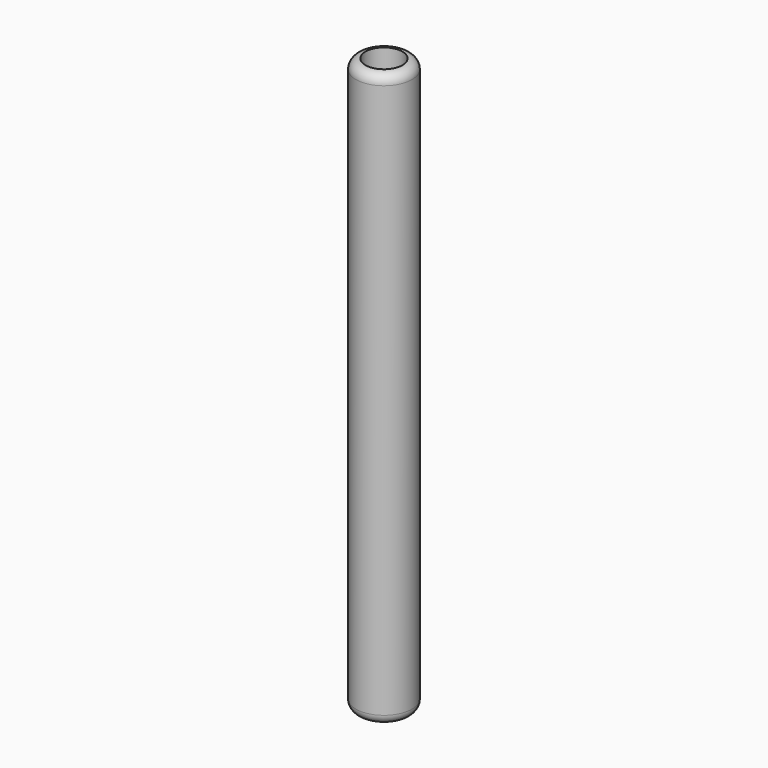
from build123d import *

# Parameters (mm, degrees)
F0_W    = 2.54
F0_H    = 152.4
F2_F1_R = 2.5399
F2_F2_R = 2.5399


# Not quite as in the source:
# - a fillet or chamfer is up to 0.001 mm smaller than in the source, because OpenCascade refuses the exact size


with BuildPart() as f1:
    # F0 (on Front) → F1 (revolve)
    with BuildSketch(Plane.XZ):
        with Locations((-6.1784988933, 0.9033400565)):
            Rectangle(F0_W, F0_H)
    revolve(axis=Axis((0, 0, -1.1060908437), (0, 0, 1)))

    # F2: fillet of radius 2.54 on 2 edges, made by hand

    # F2_f1 (radius 2.54 in the source; OpenCascade refuses exactly that, so slightly less here)
    f2_f1_edges = [f1.edges().sort_by_distance(p)[0] for p in [
        (7.4484988933, 0, 77.1033400565),
    ]]
    fillet(f2_f1_edges, radius=F2_F1_R)

    # F2_f2 (radius 2.54 in the source; OpenCascade refuses exactly that, so slightly less here)
    f2_f2_edges = [f1.edges().sort_by_distance(p)[0] for p in [
        (7.4484988933, 0, -75.2966599435),
    ]]
    fillet(f2_f2_edges, radius=F2_F2_R)


solid = f1.part
